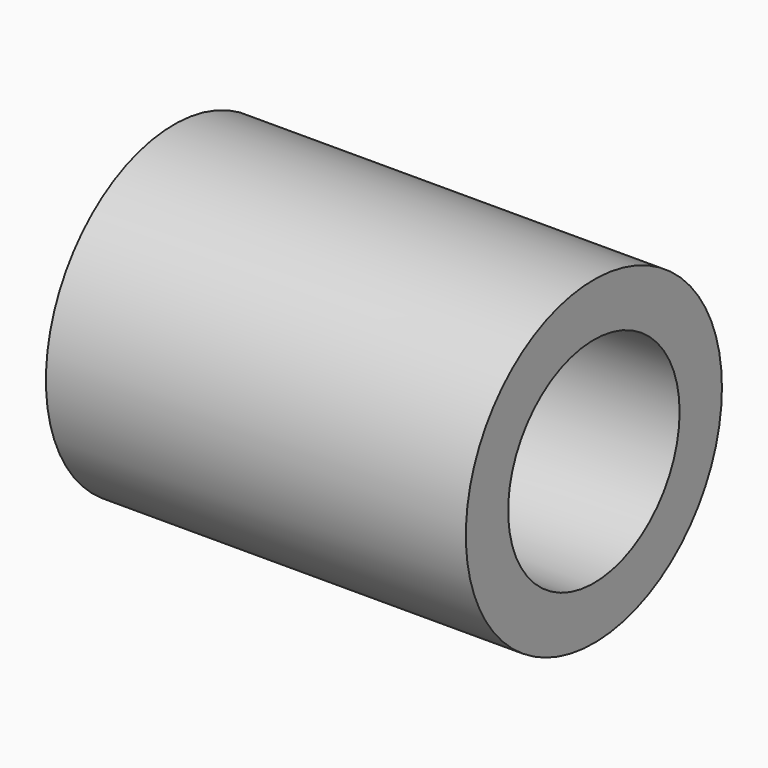
from build123d import *

# Parameters (mm, degrees)
F0_R     = 41.0468963078
F1_DEPTH = 107.696
F5_R     = 27.4816908528
F4_R     = 27.4816908528
F6_DEPTH = 76.2


# Not quite as in the source:
# - a feature of the source that left no trace in its solid (it failed there, or was rolled back) is left out


with BuildPart() as f1:
    # F0 (on Right) → F1 (new body)
    with BuildSketch(Plane.YZ):
        Circle(F0_R)
    extrude(amount=F1_DEPTH)

    # F5 (on face) + F4 (on face) → F6 (cut)
    with BuildSketch(Plane.YZ.offset(107.696)):
        Circle(F5_R)
    with BuildSketch(Plane.YZ.offset(107.696)):
        Circle(F4_R)
    extrude(amount=-F6_DEPTH, mode=Mode.SUBTRACT)


solid = f1.part
